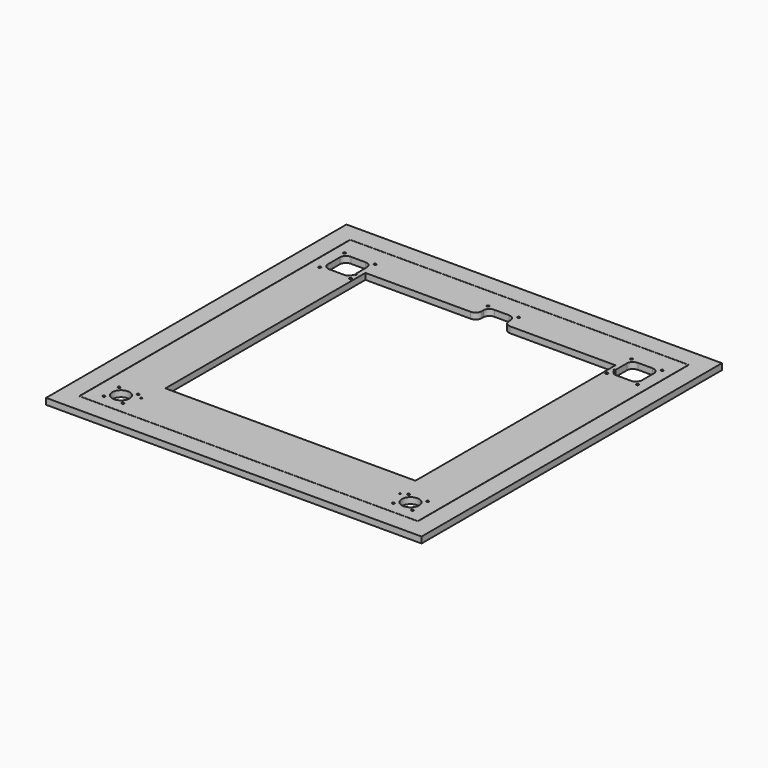
from build123d import *

# Parameters (mm, degrees)
F0_W     = 50.8
F0_H     = 50.8
F0_W_2   = 406
F0_H_2   = 406
F1_DEPTH = 10
F3_W     = 44
F3_H     = 44
F3_H_2   = 23
F3_R     = 14
F4_DEPTH = 25
F5_W     = 609.6
F5_H     = 609.6
F5_W_2   = 550
F5_H_2   = 550
F6_DEPTH = 10
F7_R     = 10
F8_D     = 4
F9_D     = 3


# Not quite as in the source:
# - a feature names something its author has since deleted; it is built from what else it names


with BuildPart() as f1:
    # F0 (on Top) → F1 (new body)
    with BuildSketch(Plane.XY):
        with Locations((249.2375, -249.2375)):
            Rectangle(F0_W, F0_H)
        Polygon((-223.8375, -274.6375), (223.8375, -274.6375), (223.8375, -223.8375), (274.6375, -223.8375), (274.6375, 223.8375), (223.8375, 223.8375), (223.8375, 274.6375), (-223.8375, 274.6375), (-223.8375, 223.8375), (-274.6375, 223.8375), (-274.6375, -223.8375), (-223.8375, -223.8375), align=None)
        with Locations((0, 13)):
            Rectangle(F0_W_2, F0_H_2, mode=Mode.SUBTRACT)
        with Locations((-249.2375, -249.2375)):
            Rectangle(F0_W, F0_H)
        with Locations((249.2375, 249.2375)):
            Rectangle(F0_W, F0_H)
        with Locations((-249.2375, 249.2375)):
            Rectangle(F0_W, F0_H)
    extrude(amount=F1_DEPTH)

    # F3 (on face) → F4 (cut)
    with BuildSketch(Plane.XY.offset(10)):
        with Locations((-233, 217)):
            Rectangle(F3_W, F3_H)
        with Locations((233, 217)):
            Rectangle(F3_W, F3_H)
        with Locations((0, 227.5)):
            Rectangle(F3_W, F3_H_2)
        with Locations((-235, -240)):
            Circle(F3_R)
        with Locations((235, -240)):
            Circle(F3_R)
    extrude(amount=-F4_DEPTH, mode=Mode.SUBTRACT)

    # F7
    f7_edges = [f1.edges().sort_by_distance(p)[0] for p in [
        (255, 195, 5),
        (255, 239, 5),
        (-22, 239, 5),
        (22, 239, 5),
        (-255, 195, 5),
        (-211, 195, 5),
        (-255, 239, 5),
        (-211, 239, 5),
        (211, 195, 5),
        (211, 239, 5),
        (22, 216, 5),
        (-22, 216, 5),
    ]]
    fillet(f7_edges, radius=F7_R)

    # F8 (through all)
    with Locations(Plane.XY.offset(10)):
        with Locations((-258, 192), (-258, 242), (-208, 242), (-208, 192), (25, 192), (25, 242), (-25, 242), (208, 192), (258, 242), (208, 242), (-25, 192), (258, 192), (-250.5, -255.5), (-250.5, -224.5), (-219.5, -224.5), (-219.5, -255.5), (250.5, -255.5), (219.5, -224.5), (219.5, -255.5), (250.5, -224.5)):
            Hole(F8_D / 2)

    # F9 (through all)
    with Locations(Plane(origin=(0, 0, 0), x_dir=(1, 0, 0), z_dir=(0, 0, -1))):
        with Locations((-210, -205), (210, -205), (210, 230), (-210, 230)):
            Hole(F9_D / 2)


with BuildPart() as f6:
    # F5 (on face) → F6 (new body)
    with BuildSketch(Plane.XY.offset(10)):
        Rectangle(F5_W, F5_H)
        Rectangle(F5_W_2, F5_H_2, mode=Mode.SUBTRACT)
    extrude(amount=-F6_DEPTH)


solid = Compound([f1.part, f6.part])
